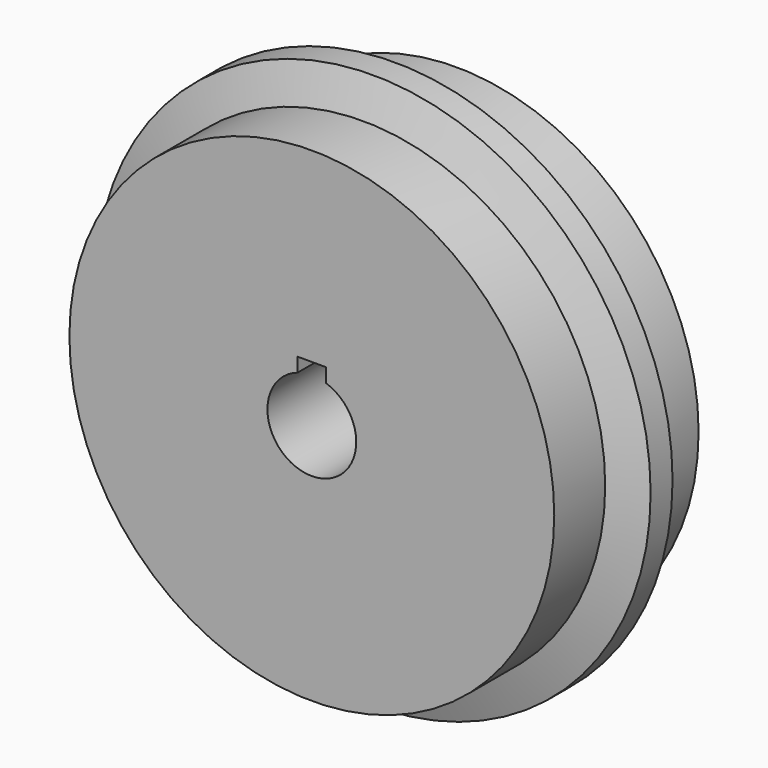
from build123d import *

# Parameters (mm, degrees)
F0_R         = 68.25
F0_R_2       = 12.5
F1_DEPTH     = 25.4
F2_W         = 8
F2_H         = 15.8
F3_DEPTH     = 50.801
F4_R         = 78.15
F4_R_2       = 20
F5_DEPTH     = 7.5
F6_S5_R      = 68.25
F6_T6_DEPTH  = 112
F6_S11_R     = 68.25
F6_T12_DEPTH = 112


# Not quite as in the source:
# - a fillet or chamfer that OpenCascade refuses, or shapes differently, is made with other operations: its cross-section is extruded or revolved along the edge and cut away or added


with BuildPart() as f1:
    # F0 (on Front) → F1 (new body, symmetric)
    with BuildSketch(Plane.XZ):
        Circle(F0_R)
        Circle(F0_R_2, mode=Mode.SUBTRACT)
    extrude(amount=F1_DEPTH, both=True)

    # F2 (on face) → F3 (cut, through all)
    with BuildSketch(Plane.XZ.offset(25.4)):
        with Locations((0, 7.9)):
            Rectangle(F2_W, F2_H)
    extrude(amount=-F3_DEPTH, mode=Mode.SUBTRACT)

    # F4 (on Front) → F5 (join, symmetric)
    with BuildSketch(Plane.XZ):
        Circle(F4_R)
        Circle(F4_R_2, mode=Mode.SUBTRACT)
    extrude(amount=F5_DEPTH, both=True)

    # F6: chamfer of 10 x 3.6397023427 on 2 edges, made by hand


with BuildPart() as f6_tool2:
    # F6_s3 → F6_t4 (revolve)
    with BuildSketch(Plane.XY):
        Polygon((78.15, -3.8602976573), (68.15, -7.5), (78.15, -7.5), align=None)
    revolve(axis=Axis((0, -7.5, 0), (0, -1, 0)))

    # F6_s5 → F6_t6 (cut, symmetric)
    with BuildSketch(Plane.XZ.offset(5.7)):
        Circle(F6_S5_R)
    extrude(amount=F6_T6_DEPTH, both=True, mode=Mode.SUBTRACT)


with BuildPart() as f1_1:
    add(f1.part)

    # F6_t1: cut F6_tool2
    add(f6_tool2.part, mode=Mode.SUBTRACT)


with BuildPart() as f6_tool8:
    # F6_s9 → F6_t10 (revolve)
    with BuildSketch(Plane.XY):
        Polygon((68.15, 7.5), (78.15, 3.8602976573), (78.15, 7.5), align=None)
    revolve(axis=Axis((0, 7.5, 0), (0, -1, 0)))

    # F6_s11 → F6_t12 (cut, symmetric)
    with BuildSketch(Plane.XZ.offset(-5.7)):
        Circle(F6_S11_R)
    extrude(amount=F6_T12_DEPTH, both=True, mode=Mode.SUBTRACT)


with BuildPart() as f1_2:
    add(f1_1.part)

    # F6_t7: cut F6_tool8
    add(f6_tool8.part, mode=Mode.SUBTRACT)


solid = f1_2.part
